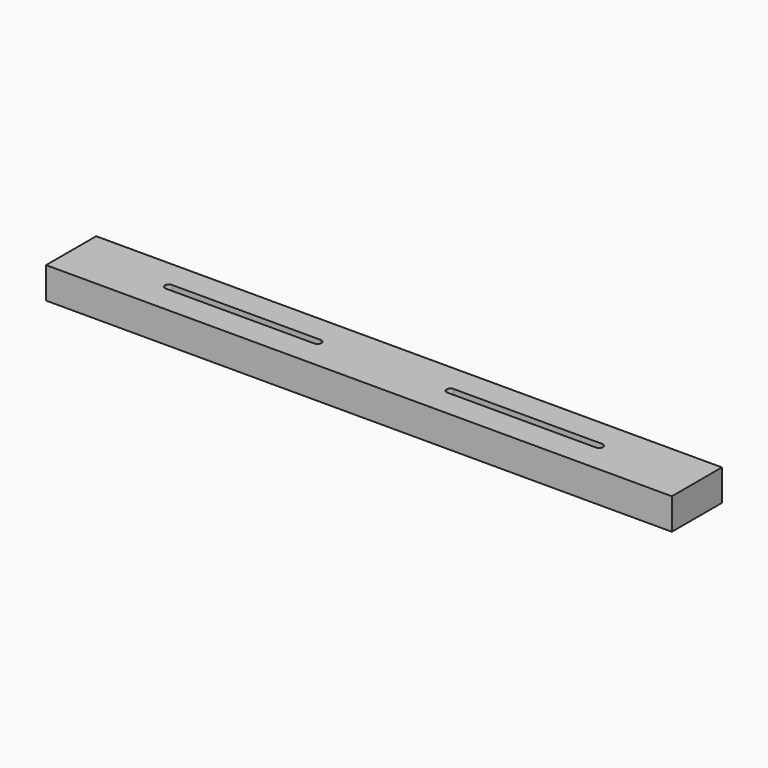
from build123d import *

# Parameters (mm, degrees)
F0_W     = 40
F0_H     = 4
F1_DEPTH = 2
F2_W     = 10
F2_H     = 0.5
F3_DEPTH = 1
F4_R     = 0.25
F5_DEPTH = 25
F6_R     = 0.24999


# Not quite as in the source:
# - a fillet or chamfer is up to 0.001 mm smaller than in the source, because OpenCascade refuses the exact size


with BuildPart() as f1:
    # F0 (on Top) → F1 (new body)
    with BuildSketch(Plane.XY):
        Rectangle(F0_W, F0_H)
    extrude(amount=F1_DEPTH)

    # F2 (on face) → F3 (cut)
    with BuildSketch(Plane.XY.offset(2)):
        with Locations((-9, 0)):
            Rectangle(F2_W, F2_H)
        with Locations((9, 0)):
            Rectangle(F2_W, F2_H)
    extrude(amount=-F3_DEPTH, mode=Mode.SUBTRACT)

    # F4 (on face) → F5 (cut)
    with BuildSketch(Plane.XY.offset(1)):
        with BuildLine():
            ThreePointArc((-13.75, -0.25), (-13.5732233047, -0.1767766953), (-13.5, 0))
            ThreePointArc((-13.5, 0), (-13.5732233047, 0.1767766953), (-13.75, 0.25))
            ThreePointArc((-13.75, 0.25), (-13.9267766953, 0.1767766953), (-14, 0))
            ThreePointArc((-14, 0), (-13.9267766953, -0.1767766953), (-13.75, -0.25))
        make_face()
        with BuildLine():
            ThreePointArc((-4, 0), (-4.0732233047, 0.1767766953), (-4.25, 0.25))
            ThreePointArc((-4.25, 0.25), (-4.5, 0), (-4.25, -0.25))
            ThreePointArc((-4.25, -0.25), (-4.0732233047, -0.1767766953), (-4, 0))
        make_face()
        with Locations((13.75, 0)):
            Circle(F4_R)
        with Locations((4.25, 0)):
            Circle(F4_R)
    extrude(amount=-F5_DEPTH, mode=Mode.SUBTRACT)

    # F6 (radius 0.25 in the source; OpenCascade refuses exactly that, so slightly less here)
    f6_edges = [f1.edges().sort_by_distance(p)[0] for p in [
        (14, 0.25, 1.5),
        (14, -0.25, 1.5),
        (4, -0.25, 1.5),
        (4, 0.25, 1.5),
        (-14, 0.25, 1.5),
        (-14, -0.25, 1.5),
        (-4, 0.25, 1.5),
        (-4, -0.25, 1.5),
    ]]
    fillet(f6_edges, radius=F6_R)


solid = f1.part
